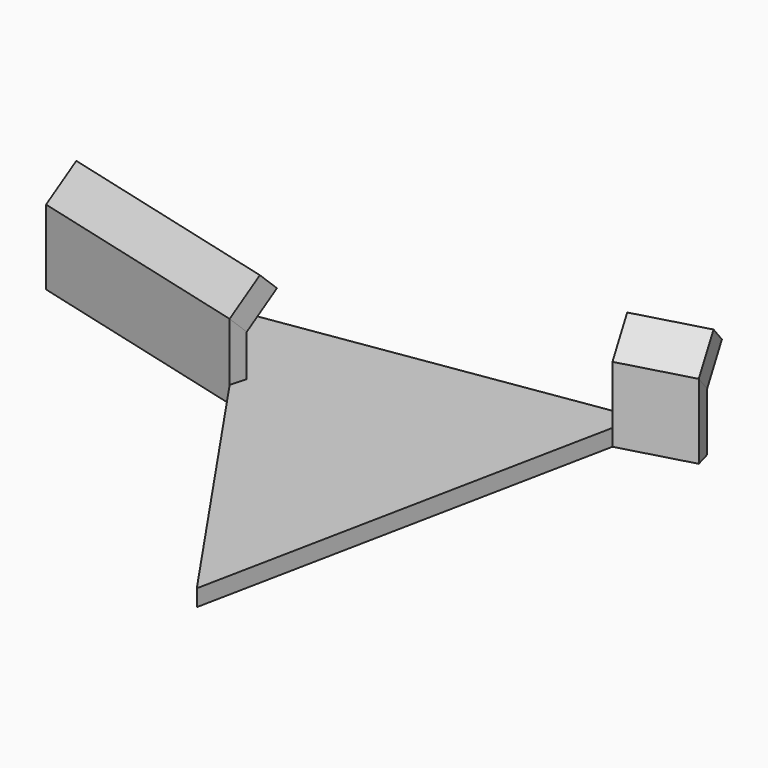
from build123d import *

# Parameters (mm, degrees)
F1_DEPTH  = 2
F3_DEPTH  = 7
F4_SIZE   = 1.99999
F6_DEPTH  = 5
F8_DEPTH  = 5
F9_R      = 2.25
F10_DEPTH = 2
F11_R     = 4.5
F12_DEPTH = 2


# Not quite as in the source:
# - a fillet or chamfer is up to 0.001 mm smaller than in the source, because OpenCascade refuses the exact size


with BuildPart() as f1:
    # F0 (on Top) → F1 (new body)
    with BuildSketch(Plane.XY):
        Polygon((-28.5105540231, 5.458955369), (-0.5105540231, -1.9337359151), (22.9272134602, -36.1708849669), (33.0351494605, 13.7129257786), (41.5351494605, 16.0733799656), (41, 18.000454187), (-28, 7.3926912842), align=None)
    extrude(amount=F1_DEPTH)

    # F2 (on face) → F3 (join)
    with BuildSketch(Plane.XY.offset(2)):
        Polygon((-28.5105540231, 5.458955369), (-0.5105540231, -1.9337359151), (0, 0), (-28, 7.3926912842), align=None)
        Polygon((32.5, 15.64), (33.0351494605, 13.7129257786), (41.5351494605, 16.0733799656), (41, 18.000454187), align=None)
    extrude(amount=F3_DEPTH)

    # F4 (size 2 in the source; OpenCascade refuses exactly that, so slightly less here)
    f4_edges = [f1.edges().sort_by_distance(p)[0] for p in [
        (-14, 3.696346, 9),
        (36.75, 16.820227, 9),
    ]]
    chamfer(f4_edges, length=F4_SIZE)

    # F5 (on face) → F6 (join)
    with BuildSketch(Plane(origin=(0.8934695404, 3.3840378515, 3.5), x_dir=(0.9835734968, -0.125470625, -0.129770176), z_dir=(0.1805081059, 0.6836788893, 0.7071067812))):
        Polygon((-1.4274719357, -7.6460659082), (-0.9083912318, -4.8656783052), (-29.3760147392, 0.4490461714), (-29.8950954431, -2.3313414316), align=None)
    extrude(amount=F6_DEPTH)

    # F7 (on face) → F8 (join)
    with BuildSketch(Plane(origin=(-1.7892109036, 6.442951854, 6.6867708388), x_dir=(0.9819378198, 0.1312802997, 0.1362483066), z_dir=(-0.1892039063, 0.6813236249, 0.7071067812))):
        Polygon((43.5762937763, 8.105378656), (34.9199411754, 6.4055834869), (35.4649344018, 3.6301587657), (44.1212870028, 5.3299539348), align=None)
    extrude(amount=F8_DEPTH)

    # F9 (on face) → F10 (join)
    with BuildSketch(Plane(origin=(0, 0, 0), x_dir=(1, 0, 0), z_dir=(0, 0, -1))):
        with Locations((16.5175747303, -7.0523503236)):
            Circle(F9_R)
    extrude(amount=F10_DEPTH)

    # F11 (on face) → F12 (join)
    with BuildSketch(Plane(origin=(0, 0, -2), x_dir=(1, 0, 0), z_dir=(0, 0, -1))):
        with Locations((16.5175747303, -7.0523503236)):
            Circle(F11_R)
    extrude(amount=F12_DEPTH)


solid = f1.part
